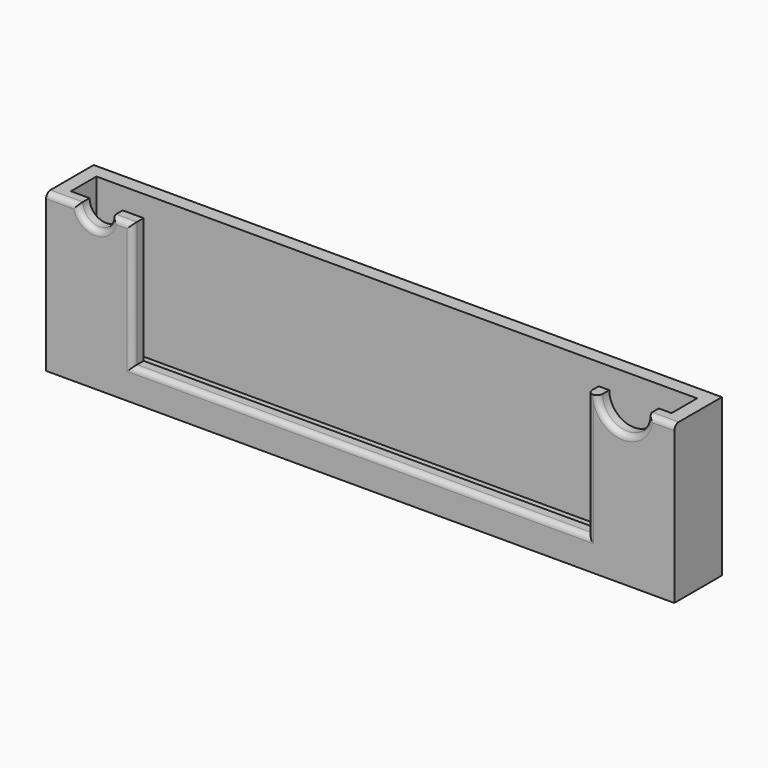
from build123d import *

# Parameters (mm, degrees)
F0_W          = 144.78
F0_H          = 13.716
F1_DEPTH      = 36.195
F2_W          = 138.43
F2_H          = 7.366
F3_DEPTH      = 33.02
F4_W          = 104.902
F4_H          = 28.956
F5_DEPTH      = 3.175
F6_W          = 25.4
F6_H          = 19.05
F7_DEPTH      = 36.195
F8_W          = 19.05
F8_H          = 19.05
F9_DEPTH      = 31.115
F11_DEPTH     = 25.4
F12_R         = 2.38125
F13_DEPTH     = 25.4
F14_R         = 9.525
F15_T1_DEPTH  = 104.902
F15_T3_DEPTH  = 13.843
F15_T5_DEPTH  = 11.176
F15_T7_DEPTH  = 12.446
F15_T9_DEPTH  = 32.131
F15_T12_ANGLE = 243.7643577336
F15_T14_ANGLE = 275.6465366004
F15_T19_DEPTH = 108.077
F15_T23_DEPTH = 32.131
F15_T30_DEPTH = 32.131
F15_T34_DEPTH = 108.077


# Not quite as in the source:
# - a fillet or chamfer that OpenCascade refuses, or shapes differently, is made with other operations: its cross-section is extruded or revolved along the edge and cut away or added


with BuildPart() as f1:
    # F0 (on Top) → F1 (new body)
    with BuildSketch(Plane.XY):
        with Locations((72.39, 6.858)):
            Rectangle(F0_W, F0_H)
    extrude(amount=F1_DEPTH)

    # F2 (on face) → F3 (cut)
    with BuildSketch(Plane.XY.offset(36.195)):
        with Locations((72.39, 6.858)):
            Rectangle(F2_W, F2_H)
    extrude(amount=-F3_DEPTH, mode=Mode.SUBTRACT)

    # F4 (on face) → F5 (cut)
    with BuildSketch(Plane.XZ):
        with BuildLine():
            ThreePointArc((7.493, 36.195), (11.303, 32.385), (15.113, 36.195))
            Line((15.113, 36.195), (7.493, 36.195))
        make_face()
        with Locations((72.39, 21.717)):
            Rectangle(F4_W, F4_H)
        with BuildLine():
            Line((138.684, 36.195), (127.254, 36.195))
            ThreePointArc((127.254, 36.195), (132.969, 30.48), (138.684, 36.195))
        make_face()
    extrude(amount=-F5_DEPTH, mode=Mode.SUBTRACT)

    # F6 (on Top) → F7 (join)
    with BuildSketch(Plane.XY):
        with Locations((72.39, 23.241)):
            Rectangle(F6_W, F6_H)
    extrude(amount=F7_DEPTH)

    # F8 (on face) → F9 (cut)
    with BuildSketch(Plane.XY.offset(36.195)):
        with Locations((72.39, 23.241)):
            Rectangle(F8_W, F8_H)
    extrude(amount=-F9_DEPTH, mode=Mode.SUBTRACT)

    # F10 (on face) → F11 (cut)
    with BuildSketch(Plane.YZ.offset(85.09)):
        Polygon((32.766, 36.195), (13.716, 36.195), (32.766, 5.08), align=None)
    extrude(amount=-F11_DEPTH, mode=Mode.SUBTRACT)

    # F12 (on face) → F13 (cut)
    with BuildSketch(Plane(origin=(0, 0, 0), x_dir=(1, 0, 0), z_dir=(0, 0, -1))):
        with Locations((72.39, -22.44725)):
            Circle(F12_R)
    extrude(amount=-F13_DEPTH, mode=Mode.SUBTRACT)

    # F14
    f14_edges = [f1.edges().sort_by_distance(p)[0] for p in [
        (141.605, 6.858, 3.175),
        (3.175, 6.858, 3.175),
    ]]
    fillet(f14_edges, radius=F14_R)

    # F15: fillet of radius 1.27 on 9 edges, made by hand

    # F15_s2 → F15_t1 (cut)
    with BuildSketch(Plane.YZ.offset(19.939)):
        with BuildLine():
            ThreePointArc((1.27, 7.239), (0.3719743879, 6.8670256121), (0, 5.969))
            Line((0, 5.969), (0, 7.239))
            Line((0, 7.239), (1.27, 7.239))
        make_face()
    extrude(amount=F15_T1_DEPTH, mode=Mode.SUBTRACT)

    # F15_s4 → F15_t3 (cut)
    with BuildSketch(Plane.YZ.offset(-3.175)):
        with BuildLine():
            ThreePointArc((1.27, 36.195), (0.3719743879, 35.8230256121), (0, 34.925))
            Line((0, 34.925), (0, 36.195))
            Line((0, 36.195), (1.27, 36.195))
        make_face()
    extrude(amount=F15_T3_DEPTH, mode=Mode.SUBTRACT)

    # F15_s6 → F15_t5 (cut)
    with BuildSketch(Plane.YZ.offset(11.938)):
        with BuildLine():
            ThreePointArc((1.27, 36.195), (0.3719743879, 35.8230256121), (0, 34.925))
            Line((0, 34.925), (0, 36.195))
            Line((0, 36.195), (1.27, 36.195))
        make_face()
    extrude(amount=F15_T5_DEPTH, mode=Mode.SUBTRACT)

    # F15_s8 → F15_t7 (cut)
    with BuildSketch(Plane.YZ.offset(135.509)):
        with BuildLine():
            ThreePointArc((1.27, 36.195), (0.3719743879, 35.8230256121), (0, 34.925))
            Line((0, 34.925), (0, 36.195))
            Line((0, 36.195), (1.27, 36.195))
        make_face()
    extrude(amount=F15_T7_DEPTH, mode=Mode.SUBTRACT)

    # F15_s10 → F15_t9 (cut)
    with BuildSketch(Plane.XY.offset(7.239)):
        with BuildLine():
            ThreePointArc((19.939, 1.27), (19.5670256121, 0.3719743879), (18.669, 0))
            Line((18.669, 0), (19.939, 0))
            Line((19.939, 0), (19.939, 1.27))
        make_face()
        with BuildLine():
            ThreePointArc((124.841, 1.27), (125.2129743879, 0.3719743879), (126.111, 0))
            Line((126.111, 0), (124.841, 0))
            Line((124.841, 0), (124.841, 1.27))
        make_face()
    extrude(amount=F15_T9_DEPTH, mode=Mode.SUBTRACT)

    # F15_s11 → F15_t12 (revolve, cut)
    with BuildSketch(Plane(origin=(53.3272604269, 0, 85.7332545483), x_dir=(0, 1, 0), z_dir=(0.5281742472, 0, 0.8491360107))):
        with BuildLine():
            ThreePointArc((1.27, -88.0764993266), (0.3719743879, -87.7045249387), (0, -86.8064993266))
            Line((0, -86.8064993266), (0, -88.0764993266))
            Line((0, -88.0764993266), (1.27, -88.0764993266))
        make_face()
    revolve(axis=Axis((132.969, 0, 36.195), (0, -1, 0)), revolution_arc=F15_T12_ANGLE, mode=Mode.SUBTRACT)

    # F15_s13 → F15_t14 (revolve, cut)
    with BuildSketch(Plane(origin=(24.217245462, 0, 21.9409429798), x_dir=(0, 1, 0), z_dir=(0.7410773266, 0, 0.6714196869))):
        with BuildLine():
            ThreePointArc((1.27, 23.0442371148), (0.3719743879, 23.4162115027), (0, 24.3142371148))
            Line((0, 24.3142371148), (0, 23.0442371148))
            Line((0, 23.0442371148), (1.27, 23.0442371148))
        make_face()
    revolve(axis=Axis((11.303, 0, 36.195), (0, -1, 0)), revolution_arc=F15_T14_ANGLE, mode=Mode.SUBTRACT)


with BuildPart() as f15_tool17:
    # F15_s18 → F15_t19 (new body)
    with BuildSketch(Plane.YZ.offset(16.764)):
        with BuildLine():
            ThreePointArc((1.27, 7.239), (0.3719743879, 6.8670256121), (0, 5.969))
            Line((0, 5.969), (0, 7.239))
            Line((0, 7.239), (1.27, 7.239))
        make_face()
    extrude(amount=F15_T19_DEPTH)

    split(bisect_by=Plane.YZ.offset(19.939), keep=Keep.BOTTOM)


with BuildPart() as f15_tool21:
    # F15_s22 → F15_t23 (new body)
    with BuildSketch(Plane.XY.offset(36.195)):
        with BuildLine():
            ThreePointArc((19.939, 1.27), (19.5670256121, 0.3719743879), (18.669, 0))
            Line((18.669, 0), (19.939, 0))
            Line((19.939, 0), (19.939, 1.27))
        make_face()
    extrude(amount=-F15_T23_DEPTH)

    split(bisect_by=Plane.XY.offset(7.239), keep=Keep.BOTTOM)


with BuildPart() as f15_tool17_1:
    add(f15_tool17.part)

    # F15_t25: intersect F15_tool21
    add(f15_tool21.part, mode=Mode.INTERSECT)


with BuildPart() as f1_1:
    add(f1.part)

    # F15_t15: cut F15_tool17
    add(f15_tool17_1.part, mode=Mode.SUBTRACT)


with BuildPart() as f15_tool28:
    # F15_s29 → F15_t30 (new body)
    with BuildSketch(Plane.XY.offset(4.064)):
        with BuildLine():
            ThreePointArc((124.841, 1.27), (125.2129743879, 0.3719743879), (126.111, 0))
            Line((126.111, 0), (124.841, 0))
            Line((124.841, 0), (124.841, 1.27))
        make_face()
    extrude(amount=F15_T30_DEPTH)

    split(bisect_by=Plane.XY.offset(7.239), keep=Keep.BOTTOM)


with BuildPart() as f15_tool32:
    # F15_s33 → F15_t34 (new body)
    with BuildSketch(Plane.YZ.offset(19.939)):
        with BuildLine():
            ThreePointArc((1.27, 7.239), (0.3719743879, 6.8670256121), (0, 5.969))
            Line((0, 5.969), (0, 7.239))
            Line((0, 7.239), (1.27, 7.239))
        make_face()
    extrude(amount=F15_T34_DEPTH)

    split(bisect_by=Plane.YZ.offset(124.841), keep=Keep.TOP)


with BuildPart() as f15_tool28_1:
    add(f15_tool28.part)

    # F15_t36: intersect F15_tool32
    add(f15_tool32.part, mode=Mode.INTERSECT)


with BuildPart() as f1_2:
    add(f1_1.part)

    # F15_t26: cut F15_tool28
    add(f15_tool28_1.part, mode=Mode.SUBTRACT)


solid = f1_2.part
